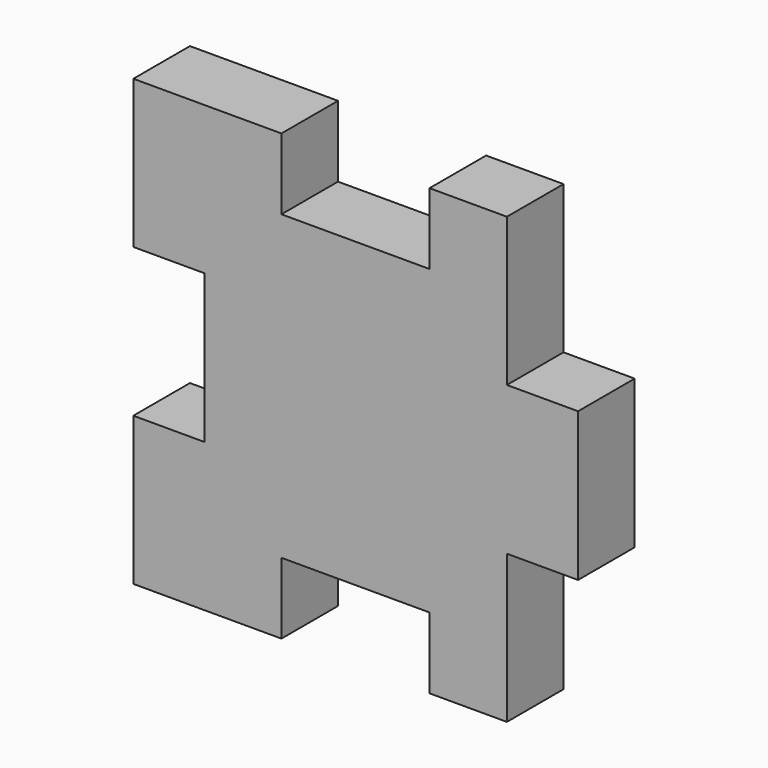
from build123d import *

# Parameters (mm, degrees)
F1_DEPTH     = 2.032
F3_TEXT_SIZE = 7.9374903895
F4_DEPTH     = 0.508


# Not quite as in the source:
# - Text() gives the source's letters only with a copy of the font that has no kerning and outlines rounded to 1/6400 em; it was checked with that copy


with BuildPart() as f1:
    # F0 (on Front) → F1 (new body)
    with BuildSketch(Plane.XZ):
        Polygon((-10.9897290399, 29.0234165891), (-10.9897290399, 26.8898165891), (-10.9897290399, 24.7562165891), (-13.0344290399, 24.7562165891), (-13.0344290399, 20.5017165891), (-8.7799290399, 20.5017165891), (-8.7799290399, 22.5464165891), (-4.5254290399, 22.5464165891), (-4.5254290399, 20.5017165891), (-2.3029290399, 20.5017165891), (-2.3029290399, 24.7562165891), (-0.2582290399, 24.7562165891), (-0.2582290399, 29.0234165891), (-2.3029290399, 29.0234165891), (-2.3029290399, 33.2779165891), (-4.5254290399, 33.2779165891), (-4.5254290399, 31.2332165891), (-8.7799290399, 31.2332165891), (-8.7799290399, 33.2779165891), (-13.0344290399, 33.2779165891), (-13.0344290399, 29.0234165891), align=None)
    extrude(amount=F1_DEPTH)

    # F3 (on offset) → F4 (cut)
    with BuildSketch(Plane.XZ.offset(4.064)):
        with Locations((-9.3099086637, 24.1504731399)):
            Text('U', F3_TEXT_SIZE, font='Open Sans', text_align=(TextAlign.LEFT, TextAlign.BOTTOM))
    extrude(amount=-F4_DEPTH, mode=Mode.SUBTRACT)


solid = f1.part
